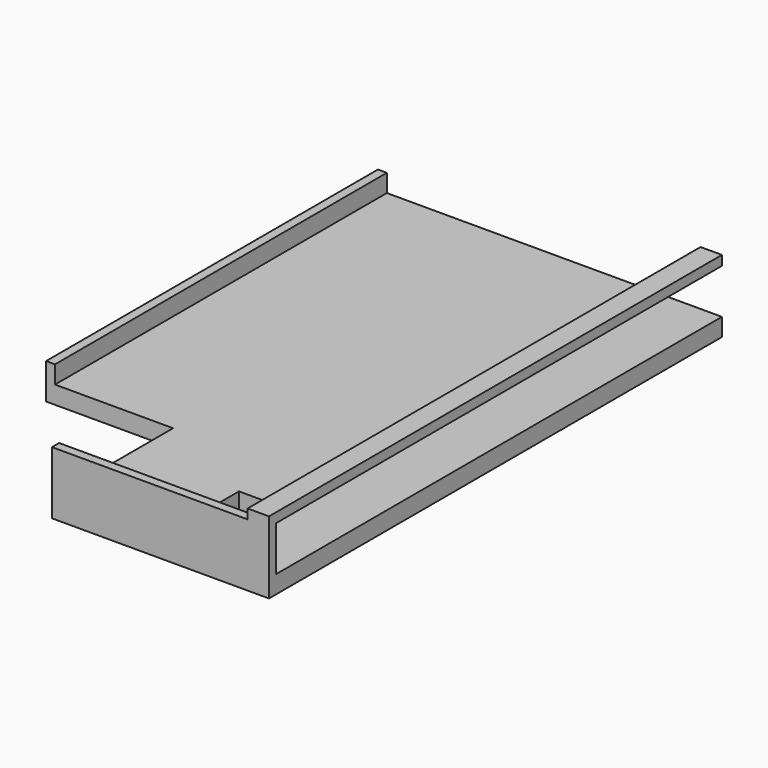
from build123d import *

# Parameters (mm, degrees)
F0_W     = 6.35
F0_H     = 13.716
F1_DEPTH = 3.175
F0_W_2   = 1.5875
F0_H_2   = 73.952875
F2_DEPTH = 6.35
F0_W_3   = 38.6812536
F0_H_3   = 1.5875
F3_DEPTH = 11.176
F7_DEPTH = 3.81


# Not quite as in the source:
# - a feature names something its author has since deleted; it is built from what else it names


with BuildPart() as f1:
    # F0 (on Top) → F1 (new body)
    with BuildSketch(Plane.XY):
        Polygon((29.8689268, -49.6764375), (29.8689268, 49.6764375), (-29.8689268, 49.6764375), (-29.8689268, -24.2764375), (-8.8123268, -24.2764375), (-8.8123268, -49.6764375), align=None)
        with Locations((13.4126732, -40.2784375)):
            Rectangle(F0_W, F0_H, mode=Mode.SUBTRACT)
    extrude(amount=F1_DEPTH)

    # F0 (on Top) → F2 (join)
    with BuildSketch(Plane.XY):
        with Locations((-30.6626768, 12.7)):
            Rectangle(F0_W_2, F0_H_2)
    extrude(amount=F2_DEPTH)

    # F0 (on Top) → F3 (join)
    with BuildSketch(Plane.XY):
        with Locations((10.5283, -50.4701875)):
            Rectangle(F0_W_3, F0_H_3)
    extrude(amount=F3_DEPTH)

    # F6 (on face) → F7 (join)
    with BuildSketch(Plane.YZ.offset(29.8689268)):
        Polygon((-51.2639375, 12.8905), (-51.2639375, 11.176), (-49.6764375, 11.176), (49.6764375, 11.176), (49.6764375, 12.8905), align=None)
    extrude(amount=-F7_DEPTH)


solid = f1.part
